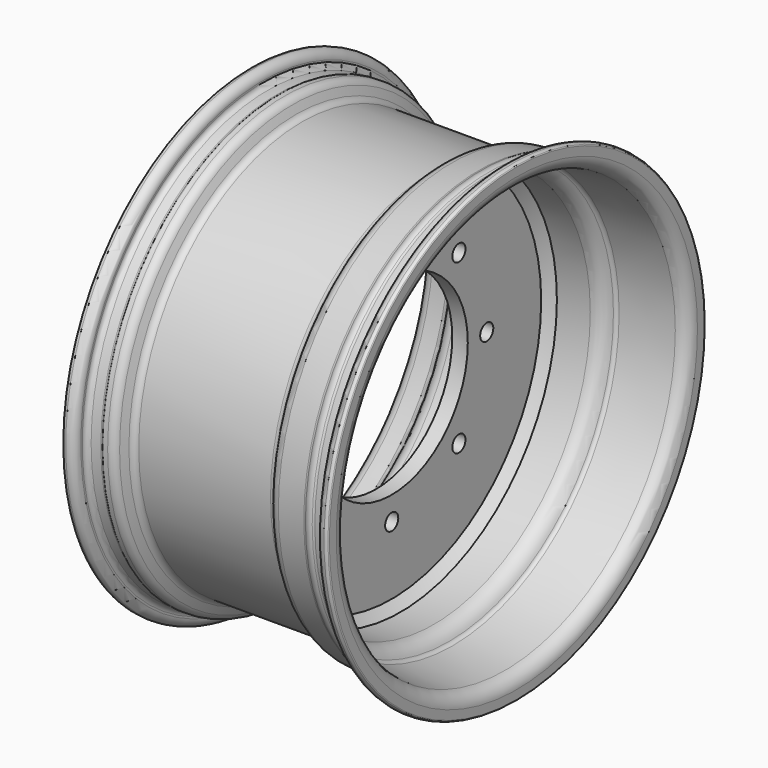
from build123d import *

# Parameters (mm, degrees)
F2_SCALE        = 2
F4_D            = 19
F4_COPIES_COUNT = 8


# Not quite as in the source:
# - ends of sketch curves that miss each other by under 0.0002 mm in the source are joined
# - a pattern or mirror of a feature is missing from the dataset's text; its kind, count and spacing are read off the source's solid


with BuildPart() as f1:
    # F0 (on Top) → F1 (revolve)
    with BuildSketch(Plane.XY):
        with BuildLine():
            Line((-69.8283927139, 130.950002), (-69.8283927139, 131.999997))
            ThreePointArc((-69.8283927139, 131.999997), (-71.2489204318, 135.4294702822), (-74.6783937139, 136.849998))
            ThreePointArc((-74.6783937139, 136.849998), (-75.6366511648, 136.703145556), (-76.50695947, 136.2760786497))
            ThreePointArc((-76.50695947, 136.2760786497), (-76.7431968016, 136.0077812035), (-76.8283927139, 135.660602))
            Line((-76.8283927139, 135.660602), (-76.8283927139, 130.666806))
            ThreePointArc((-76.8283927139, 130.666806), (-74.8579716468, 125.5998817301), (-69.9820616402, 123.195348843))
            Line((-69.9820616402, 123.195348843), (-60.4470947139, 122.361152))
            ThreePointArc((-60.4470947139, 122.361152), (-57.5619219055, 121.268055358), (-55.6730463485, 118.8285407436))
            ThreePointArc((-55.6730463485, 118.8285407436), (-52.3611274066, 114.7386622182), (-47.3283917139, 113.199999))
            Line((-47.3283917139, 113.199999), (-9.4533907139, 113.2))
            Line((-9.4533907139, 113.2), (-4.5000098646, 113.2))
            Line((-4.5000098646, 113.2), (4.4999901354, 113.2))
            Line((4.4999901354, 113.2), (9.5466092861, 113.2))
            Line((9.5466092861, 113.2), (28.8601402861, 113.2))
            ThreePointArc((28.8601402861, 113.2), (34.1166063672, 114.7867432509), (37.6171377565, 119.0169288021))
            ThreePointArc((37.6171377565, 119.0169288021), (38.4488135479, 120.0678119715), (39.70372129, 120.5381809556))
            Line((39.70372129, 120.5381809556), (70.0752792861, 123.195348))
            ThreePointArc((70.0752792861, 123.195348), (74.951189219, 125.5998817301), (76.9216092861, 130.666806))
            Line((76.9216092861, 130.666806), (76.9216102861, 135.660602))
            ThreePointArc((76.9216102861, 135.660602), (76.8364143738, 136.0077812035), (76.600177533, 136.2760793546))
            ThreePointArc((76.600177533, 136.2760793546), (75.7298687369, 136.703145556), (74.7716112861, 136.849997))
            ThreePointArc((74.7716112861, 136.849997), (71.3421380039, 135.4294702822), (69.9216102861, 131.999997))
            Line((69.9216102861, 131.999997), (69.9216102861, 130.950002))
            ThreePointArc((69.9216102861, 130.950002), (69.1334468957, 128.923223416), (67.1830752901, 127.9614099543))
            Line((67.1830752901, 127.9614099543), (62.0415972861, 127.511589))
            ThreePointArc((62.0415972861, 127.511589), (61.3420921388, 127.5323313866), (60.6664211665, 127.714557701))
            ThreePointArc((60.6664211665, 127.714557701), (58.5119771245, 128.0325485601), (56.4454811465, 127.3452772251))
            ThreePointArc((56.4454811465, 127.3452772251), (55.8117185261, 127.0484907088), (55.1264412588, 126.9066023119))
            Line((55.1264412588, 126.9066023119), (39.3317542861, 125.524743))
            ThreePointArc((39.3317542861, 125.524743), (35.565502201, 124.1125085278), (33.0705397086, 120.9574772425))
            ThreePointArc((33.0705397086, 120.9574772425), (31.4124577957, 118.9522425502), (28.9216092861, 118.199995))
            Line((28.9216092861, 118.199995), (-47.3283917139, 118.199995))
            ThreePointArc((-47.3283917139, 118.199995), (-49.5651640292, 118.8838463257), (-51.0371272461, 120.701572189))
            Line((-51.0371272461, 120.701572189), (-52.8412107139, 125.166847))
            ThreePointArc((-52.8412107139, 125.166847), (-54.6259688487, 127.3708322029), (-57.3380537139, 128.199992))
            Line((-57.3380537139, 128.199992), (-60.0783917139, 128.199993))
            ThreePointArc((-60.0783917139, 128.199993), (-60.3748925736, 128.138899496), (-60.6230889783, 127.9655682503))
            ThreePointArc((-60.6230889783, 127.9655682503), (-61.1801374973, 127.5943217232), (-61.8432187446, 127.5023946498))
            Line((-61.8432187446, 127.5023946498), (-67.0898577139, 127.96141))
            ThreePointArc((-67.0898577139, 127.96141), (-69.0402293235, 128.923223416), (-69.8283927139, 130.950002))
        make_face()
        Polygon((-4.5000098646, 113.2), (-9.4533907139, 113.2), (-4.5000098646, 108.2466171506), align=None)
        Polygon((4.4999901354, 113.2), (-4.5000098646, 113.2), (-4.5000098646, 108.2466171506), (-4.5000098646, 55.05), (4.4999901354, 55.05), (4.4999901354, 108.1533788494), align=None)
        Polygon((9.5466092861, 113.2), (4.4999901354, 113.2), (4.4999901354, 108.1533788494), align=None)
    revolve(axis=Axis((-9.8646e-06, 0, 0), (1, 0, 0)))


with BuildPart() as f1_1:
    # F2: moved
    add(f1.part.scale(F2_SCALE))

    # F4 (through all)
    with Locations(Plane.YZ.offset(8.9999802709)):
        with Locations((0, 137.5)):
            f4 = Hole(F4_D / 2)

    # F4_copies: F4 ×8 about axis
    f4_copies_axis = Axis((0, 0, 0), (1, 0, 0))
    for i in range(1, F4_COPIES_COUNT):
        add(f4.rotate(f4_copies_axis, i * 360 / F4_COPIES_COUNT), mode=Mode.SUBTRACT)


solid = f1_1.part
